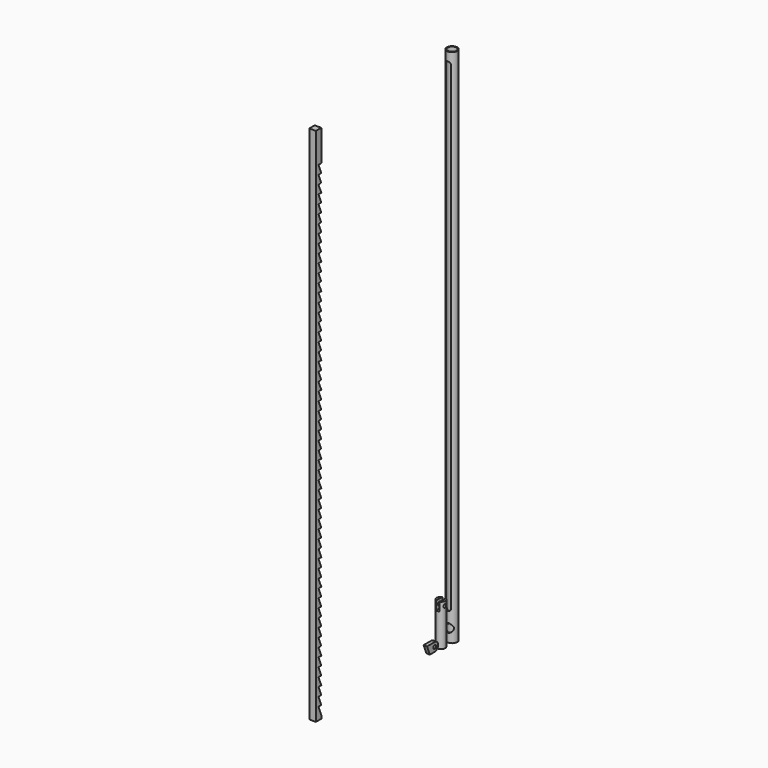
from build123d import *

# Parameters (mm, degrees)
F0_R           = 3
F0_R_2         = 2.5
F1_DEPTH       = 300
F3_DEPTH       = 25
F4_D           = 5
F4_DEPTH       = 2
F4_START       = 1.3416877
F4_TIP         = 1.5021515476
F6_DEPTH       = 2
F7_DEPTH       = 2
F8_R           = 2.45
F9_DEPTH       = 24
F10_W          = 2
F10_H          = 7.7706239607
F11_DEPTH      = 5
F12_R          = 1
F13_DEPTH      = 25
F13_DEPTH_BACK = 25
F14_W          = 2
F14_H          = 8
F15_DEPTH      = 5
F18_R          = 2.49999
F19_D          = 2
F20_SIZE2      = 4.99999
F20_SIZE       = 1.99999
F22_DEPTH      = 1.9
F22_DEPTH_BACK = 1.9


# Not quite as in the source:
# - a fillet or chamfer is up to 0.001 mm smaller than in the source, because OpenCascade refuses the exact size


with BuildPart() as f1:
    # F0 (on Top) → F1 (new body)
    with BuildSketch(Plane.XY):
        with Locations((0, 3)):
            Circle(F0_R)
        with Locations((0, 3)):
            Circle(F0_R_2, mode=Mode.SUBTRACT)
    extrude(amount=F1_DEPTH)

    # F0 (on Top) → F3 (cut)
    with BuildSketch(Plane.XY):
        with Locations((0, 3)):
            Circle(F0_R)
        with Locations((0, 3)):
            Circle(F0_R_2, mode=Mode.SUBTRACT)
    extrude(amount=-F3_DEPTH, mode=Mode.SUBTRACT)

    # F4
    # its depths count from where the whole tool has entered the part; down to there all is cleared
    with Locations(Plane.XZ.offset(-F4_START)):
        with Locations((0, 7.5)):
            Hole(F4_D / 2, depth=F4_DEPTH)
            with Locations((0, 0, -(F4_DEPTH + F4_TIP / 2))):  # 118° drill point
                Cone(0, F4_D / 2, F4_TIP, mode=Mode.SUBTRACT)

    # F2 (on Front) + F5 (on face) → F6 (cut)
    with BuildSketch(Plane.XZ):
        with BuildLine():
            Line((0, 19), (0, 16))
            ThreePointArc((0, 16), (1.0606601718, 16.4393398282), (1.5, 17.5))
            ThreePointArc((1.5, 17.5), (1.0606601718, 18.5606601718), (0, 19))
        make_face()
        with BuildLine():
            ThreePointArc((0, 19), (-1.5, 17.5), (0, 16))
            Line((0, 16), (0, 19))
        make_face()
    with BuildSketch(Plane.XZ):
        with BuildLine():
            Line((-1.4981685921, 17.5741004028), (-1.4981685921, 17.4258995972))
            ThreePointArc((-1.4981685921, 17.4258995972), (-1.0341299231, 16.4134571789), (0, 16))
            Line((0, 16), (0, 19))
            ThreePointArc((0, 19), (-1.0341299231, 18.5865428211), (-1.4981685921, 17.5741004028))
        make_face()
    extrude(amount=F6_DEPTH, mode=Mode.SUBTRACT)

    # F2 (on Front) + F5 (on face) → F7 (cut)
    with BuildSketch(Plane.XZ):
        with BuildLine():
            ThreePointArc((0, 295), (-1.5, 293.5), (0, 292))
            Line((0, 292), (0, 295))
        make_face()
        with BuildLine():
            Line((0, 295), (0, 292))
            ThreePointArc((0, 292), (1.0606601718, 292.4393398282), (1.5, 293.5))
            ThreePointArc((1.5, 293.5), (1.0606601718, 294.5606601718), (0, 295))
        make_face()
        with BuildLine():
            ThreePointArc((0, 19), (-1.5, 17.5), (0, 16))
            Line((0, 16), (0, 19))
        make_face()
        with BuildLine():
            Line((0, 19), (0, 16))
            ThreePointArc((0, 16), (1.0606601718, 16.4393398282), (1.5, 17.5))
            ThreePointArc((1.5, 17.5), (1.0606601718, 18.5606601718), (0, 19))
        make_face()
    with BuildSketch(Plane.XZ):
        with BuildLine():
            Line((-1.4981685921, 17.5741004028), (-1.4981685921, 17.4258995972))
            ThreePointArc((-1.4981685921, 17.4258995972), (-1.0341299231, 16.4134571789), (0, 16))
            Line((0, 16), (0, 19))
            ThreePointArc((0, 19), (-1.0341299231, 18.5865428211), (-1.4981685921, 17.5741004028))
        make_face()
        with BuildLine():
            Line((0, 19), (0, 16))
            ThreePointArc((0, 16), (1.0341299231, 16.4134571789), (1.4981685921, 17.4258995972))
            Line((1.4981685921, 17.4258995972), (1.4981685921, 17.5741004028))
            ThreePointArc((1.4981685921, 17.5741004028), (1.0341299231, 18.5865428211), (0, 19))
        make_face()
        with BuildLine():
            Line((-1.4981685921, 293.4258995972), (-1.4981685921, 17.5741004028))
            ThreePointArc((-1.4981685921, 17.5741004028), (-1.0341299231, 18.5865428211), (0, 19))
            Line((0, 19), (0, 292))
            ThreePointArc((0, 292), (-1.0341299231, 292.4134571789), (-1.4981685921, 293.4258995972))
        make_face()
        with BuildLine():
            Line((0, 292), (0, 19))
            ThreePointArc((0, 19), (1.0341299231, 18.5865428211), (1.4981685921, 17.5741004028))
            Line((1.4981685921, 17.5741004028), (1.4981685921, 293.4258995972))
            ThreePointArc((1.4981685921, 293.4258995972), (1.0341299231, 292.4134571789), (0, 292))
        make_face()
    extrude(amount=-F7_DEPTH, mode=Mode.SUBTRACT)


with BuildPart() as f9:
    # F8 (on Top) → F9 (new body)
    with BuildSketch(Plane.XY):
        with Locations((0, -5.0555539014)):
            Circle(F8_R)
    extrude(amount=F9_DEPTH)

    # F10 (on face) → F11 (cut)
    with BuildSketch(Plane.XY.offset(24)):
        with Locations((0, -5.0555539014)):
            Rectangle(F10_W, F10_H)
    extrude(amount=-F11_DEPTH, mode=Mode.SUBTRACT)

    # F12 (on Right) → F13 (cut, two sides)
    with BuildSketch(Plane.YZ) as f13_sk:
        with Locations((-5.0555539014, 21.5)):
            Circle(F12_R)
    extrude(amount=F13_DEPTH, mode=Mode.SUBTRACT)
    extrude(f13_sk.sketch, amount=-F13_DEPTH_BACK, mode=Mode.SUBTRACT)


with BuildPart() as f15:
    # F14 (on Top) → F15 (new body)
    with BuildSketch(Plane.XY):
        with Locations((0, -12.3077967234)):
            Rectangle(F14_W, F14_H)
    extrude(amount=F15_DEPTH)

    # F18 (radius 2.5 in the source; OpenCascade refuses exactly that, so slightly less here)
    f18_edges = [f15.edges().sort_by_distance(p)[0] for p in [
        (0, -8.307797, 0),
        (0, -8.307797, 5),
    ]]
    fillet(f18_edges, radius=F18_R)

    # F19 (through all)
    with Locations(Plane.YZ.offset(1)):
        with Locations((-10.8077967234, 2.5)):
            Hole(F19_D / 2)

    # F20 (size 2 and 5 in the source; OpenCascade refuses exactly that, so slightly less here)
    f20_edges = [f15.edges().sort_by_distance(p)[0] for p in [
        (0, -16.307797, 0),
    ]]
    f20_side = f15.faces().sort_by_distance((0, -13.557792, 0))[0]
    chamfer(f20_edges, length=F20_SIZE, length2=F20_SIZE2, reference=f20_side)


with BuildPart() as f22:
    # F21 (on Right) → F22 (new body, two sides)
    with BuildSketch(Plane.YZ) as f22_sk:
        Polygon((-97.5489613374, 300), (-97.5489613374, 0), (-93.6489613374, 0), (-93.6489613374, 2), (-95.6489613374, 7), (-93.6489613374, 7), (-95.6489613374, 12), (-93.6489613374, 12), (-95.6489613374, 17), (-93.6489613374, 17), (-95.6489613374, 22), (-93.6489613374, 22), (-95.6489613374, 27), (-93.6489613374, 27), (-95.6489613374, 32), (-93.6489613374, 32), (-95.6489613374, 37), (-93.6489613374, 37), (-95.6489613374, 42), (-93.6489613374, 42), (-95.6489613374, 47), (-93.6489613374, 47), (-95.6489613374, 52), (-93.6489613374, 52), (-95.6489613374, 57), (-93.6489613374, 57), (-95.6489613374, 62), (-93.6489613374, 62), (-95.6489613374, 67), (-93.6489613374, 67), (-95.6489613374, 72), (-93.6489613374, 72), (-95.6489613374, 77), (-93.6489613374, 77), (-95.6489613374, 82), (-93.6489613374, 82), (-95.6489613374, 87), (-93.6489613374, 87), (-95.6489613374, 92), (-93.6489613374, 92), (-95.6489613374, 97), (-93.6489613374, 97), (-95.6489613374, 102), (-93.6489613374, 102), (-95.6489613374, 107), (-93.6489613374, 107), (-95.6489613374, 112), (-93.6489613374, 112), (-95.6489613374, 117), (-93.6489613374, 117), (-95.6489613374, 122), (-93.6489613374, 122), (-95.6489613374, 127), (-93.6489613374, 127), (-95.6489613374, 132), (-93.6489613374, 132), (-95.6489613374, 137), (-93.6489613374, 137), (-95.6489613374, 142), (-93.6489613374, 142), (-95.6489613374, 147), (-93.6489613374, 147), (-95.6489613374, 152), (-93.6489613374, 152), (-95.6489613374, 157), (-93.6489613374, 157), (-95.6489613374, 162), (-93.6489613374, 162), (-95.6489613374, 167), (-93.6489613374, 167), (-95.6489613374, 172), (-93.6489613374, 172), (-95.6489613374, 177), (-93.6489613374, 177), (-95.6489613374, 182), (-93.6489613374, 182), (-95.6489613374, 187), (-93.6489613374, 187), (-95.6489613374, 192), (-93.6489613374, 192), (-95.6489613374, 197), (-93.6489613374, 197), (-95.6489613374, 202), (-93.6489613374, 202), (-95.6489613374, 207), (-93.6489613374, 207), (-95.6489613374, 212), (-93.6489613374, 212), (-95.6489613374, 217), (-93.6489613374, 217), (-95.6489613374, 222), (-93.6489613374, 222), (-95.6489613374, 227), (-93.6489613374, 227), (-95.6489613374, 232), (-93.6489613374, 232), (-95.6489613374, 237), (-93.6489613374, 237), (-95.6489613374, 242), (-93.6489613374, 242), (-95.6489613374, 247), (-93.6489613374, 247), (-95.6489613374, 252), (-93.6489613374, 252), (-95.6489613374, 257), (-93.6489613374, 257), (-95.6489613374, 262), (-93.6489613374, 262), (-95.6489613374, 267), (-93.6489613374, 267), (-95.6489613374, 272), (-93.6489613374, 272), (-95.6489613374, 277), (-93.6489613374, 277), (-95.6489613374, 282), (-93.6489613374, 282), (-93.6489613374, 300), align=None)
    extrude(amount=F22_DEPTH)
    extrude(f22_sk.sketch, amount=-F22_DEPTH_BACK)


solid = Compound([f1.part, f9.part, f15.part, f22.part])
